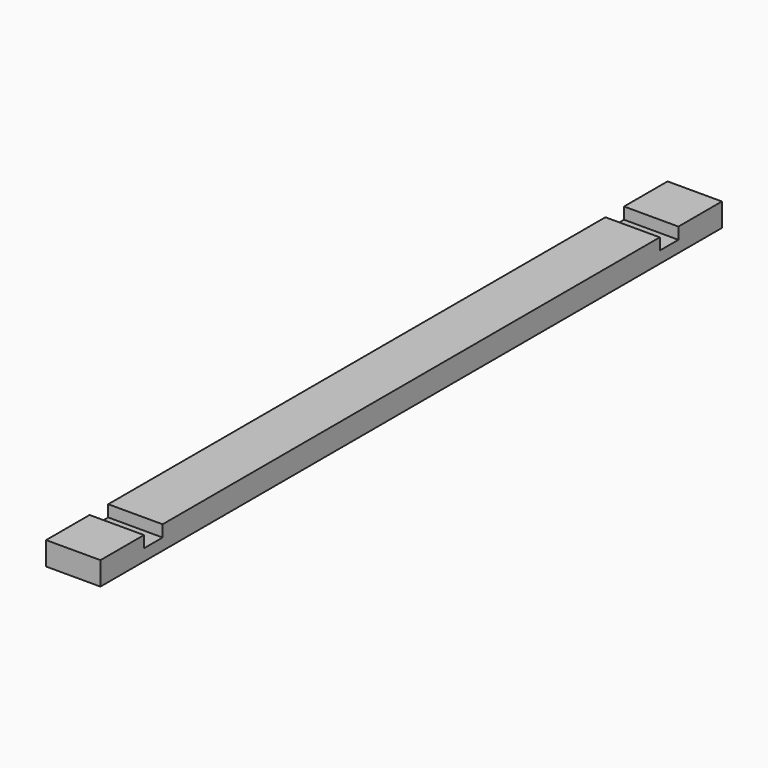
from build123d import *

# Parameters (mm, degrees)
F0_W     = 88.9
F0_H     = 38.1
F1_DEPTH = 635
F2_W     = 88.9
F2_H     = 38.1
F3_DEPTH = 19.05


# Not quite as in the source:
# - a length typed as a fraction of an inch, garbled in the dataset ("3 / 203.2 mm" for 3/8 in), is restored


with BuildPart() as f1:
    # F0 (on Front) → F1 (new body, symmetric)
    with BuildSketch(Plane.XZ):
        Rectangle(F0_W, F0_H)
    extrude(amount=F1_DEPTH, both=True)

    # F2 (on face) → F3 (cut)
    with BuildSketch(Plane.XY.offset(19.05)):
        with Locations((0, 527.05)):
            Rectangle(F2_W, F2_H)
        with Locations((0, -527.05)):
            Rectangle(F2_W, F2_H)
    extrude(amount=-F3_DEPTH, mode=Mode.SUBTRACT)


solid = f1.part
